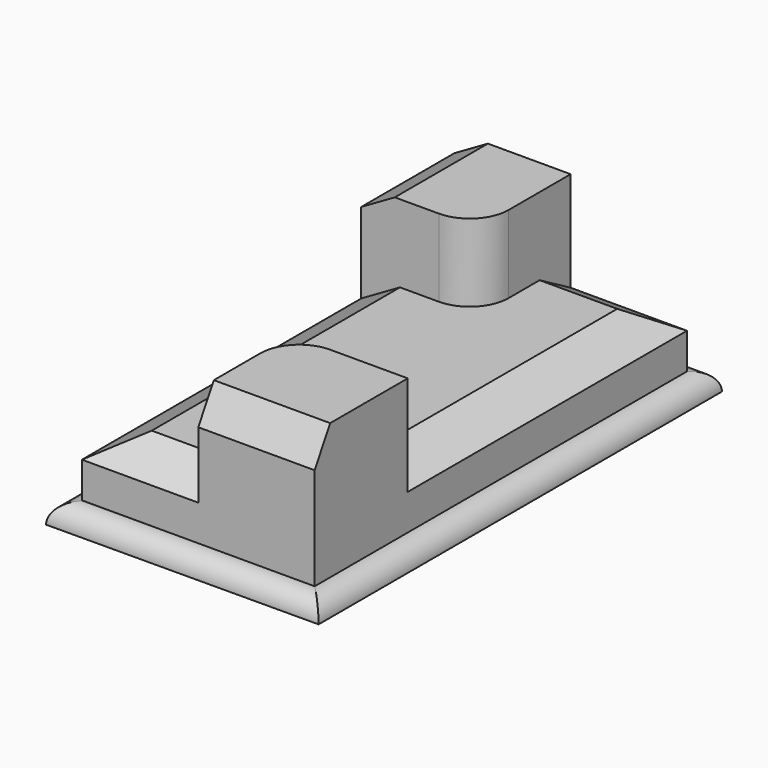
from build123d import *

# Parameters (mm, degrees)
F1_DEPTH   = 6.35
F2_DEPTH   = 25.4
F3_DEPTH   = 50.8
F4_SIZE2   = 10.9985226281
F4_SIZE    = 6.35
F4_2_SIZE2 = 10.9985226281
F4_2_SIZE  = 6.35
F5_SIZE2   = 7.3323484187
F5_SIZE    = 12.7
F6_R       = 6.34999


# Not quite as in the source:
# - a fillet or chamfer is up to 0.001 mm smaller than in the source, because OpenCascade refuses the exact size


with BuildPart() as f1:
    # F0 (on Top) → F1 (new body)
    with BuildSketch(Plane.XY):
        Polygon((-50.1812659204, 67.9668266764), (-50.1812659204, -97.5199052306), (38.7187340796, -97.1034997316), (38.7187340796, 67.9668266764), align=None)
        Polygon((-5.7312659204, -90.7831733236), (-43.8312659204, -90.7831733236), (-43.8312659204, 23.5168266764), (-43.8312659204, 61.6168266764), (-5.7312659204, 61.6168266764), (32.3687340796, 61.6168266764), (32.3687340796, -52.6831733236), (32.3687340796, -90.7831733236), align=None, mode=Mode.SUBTRACT)
    extrude(amount=F1_DEPTH)

    # F0 (on Top) → F2 (join)
    with BuildSketch(Plane.XY):
        with BuildLine():
            Line((-43.8312659204, 23.5168266764), (-43.8312659204, -90.7831733236))
            Line((-43.8312659204, -90.7831733236), (-5.7312659204, -90.7831733236))
            Line((-5.7312659204, -90.7831733236), (-5.7312659204, -65.3831733236))
            ThreePointArc((-5.7312659204, -65.3831733236), (-2.0115220415, -56.4029172025), (6.9687340796, -52.6831733236))
            Line((6.9687340796, -52.6831733236), (32.3687340796, -52.6831733236))
            Line((32.3687340796, -52.6831733236), (32.3687340796, 61.6168266764))
            Line((32.3687340796, 61.6168266764), (-5.7312659204, 61.6168266764))
            Line((-5.7312659204, 61.6168266764), (-5.7312659204, 36.2168266764))
            ThreePointArc((-5.7312659204, 36.2168266764), (-9.4510097993, 27.2365705553), (-18.4312659204, 23.5168266764))
            Line((-18.4312659204, 23.5168266764), (-43.8312659204, 23.5168266764))
        make_face()
    extrude(amount=F2_DEPTH)

    # F0 (on Top) → F3 (join)
    with BuildSketch(Plane.XY):
        with BuildLine():
            Line((-43.8312659204, 61.6168266764), (-43.8312659204, 23.5168266764))
            Line((-43.8312659204, 23.5168266764), (-18.4312659204, 23.5168266764))
            ThreePointArc((-18.4312659204, 23.5168266764), (-9.4510097993, 27.2365705553), (-5.7312659204, 36.2168266764))
            Line((-5.7312659204, 36.2168266764), (-5.7312659204, 61.6168266764))
            Line((-5.7312659204, 61.6168266764), (-43.8312659204, 61.6168266764))
        make_face()
        with BuildLine():
            Line((-5.7312659204, -65.3831733236), (-5.7312659204, -90.7831733236))
            Line((-5.7312659204, -90.7831733236), (32.3687340796, -90.7831733236))
            Line((32.3687340796, -90.7831733236), (32.3687340796, -52.6831733236))
            Line((32.3687340796, -52.6831733236), (6.9687340796, -52.6831733236))
            ThreePointArc((6.9687340796, -52.6831733236), (-2.0115220415, -56.4029172025), (-5.7312659204, -65.3831733236))
        make_face()
    extrude(amount=F3_DEPTH)

    # F4
    f4_edges = [f1.edges().sort_by_distance(p)[0] for p in [
        (13.318734, -90.783173, 50.8),
    ]]
    f4_side = f1.faces().sort_by_distance((13.714776, -72.129216, 50.8))[0]
    chamfer(f4_edges, length=F4_SIZE, length2=F4_SIZE2, reference=f4_side)

    # F4#2
    f4_2_edges = [f1.edges().sort_by_distance(p)[0] for p in [
        (-43.831266, 42.566827, 50.8),
    ]]
    f4_2_side = f1.faces().sort_by_distance((-43.831266, -0.295673, 21.43125))[0]
    chamfer(f4_2_edges, length=F4_2_SIZE, length2=F4_2_SIZE2, reference=f4_2_side)

    # F5
    f5_edges = [f1.edges().sort_by_distance(p)[0] for p in [
        (32.368734, 4.466827, 25.4),
        (-24.781266, -90.783173, 25.4),
        (-43.831266, -33.633173, 25.4),
        (13.318734, 61.616827, 25.4),
    ]]
    f5_side = f1.faces().sort_by_distance((-5.731266, -14.583173, 25.4))[0]
    chamfer(f5_edges, length=F5_SIZE, length2=F5_SIZE2, reference=f5_side)

    # F6 (radius 6.35 in the source; OpenCascade refuses exactly that, so slightly less here)
    f6_edges = [f1.edges().sort_by_distance(p)[0] for p in [
        (38.718734, -14.568337, 6.35),
        (-5.731266, -97.311702, 6.35),
        (-5.731266, 67.966827, 6.35),
        (-50.181266, -14.776539, 6.35),
    ]]
    fillet(f6_edges, radius=F6_R)


solid = f1.part
